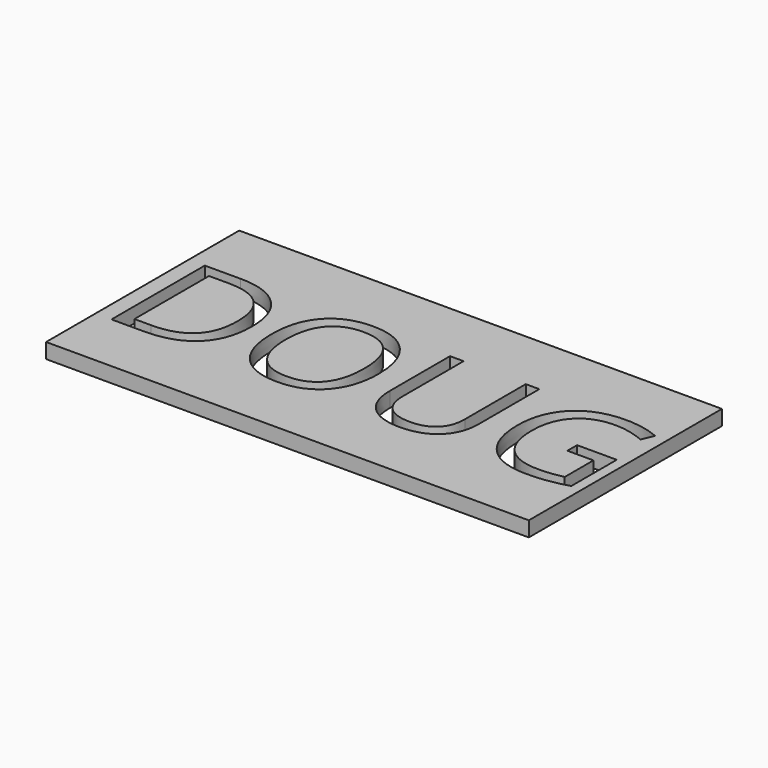
from build123d import *

# Parameters (mm, degrees)
F0_W         = 101.6
F0_H         = 50.8
F1_DEPTH     = 3.175
F2_TEXT_SIZE = 34.3947622777
F3_DEPTH     = 25.4


# Not quite as in the source:
# - Text() gives the source's letters only with a copy of the font that has no kerning and outlines rounded to 1/6400 em; it was checked with that copy


with BuildPart() as f1:
    # F0 (on Top) → F1 (new body)
    with BuildSketch(Plane.XY):
        with Locations((50.8, 25.4)):
            Rectangle(F0_W, F0_H)
    extrude(amount=F1_DEPTH)

    # F2 (on face) → F3 (cut)
    with BuildSketch(Plane.XY.offset(3.175)):
        with Locations((0, 12.9852764481)):
            Text('DOUG', F2_TEXT_SIZE, font='Open Sans', text_align=(TextAlign.LEFT, TextAlign.BOTTOM))
    extrude(amount=-F3_DEPTH, mode=Mode.SUBTRACT)


solid = f1.part
